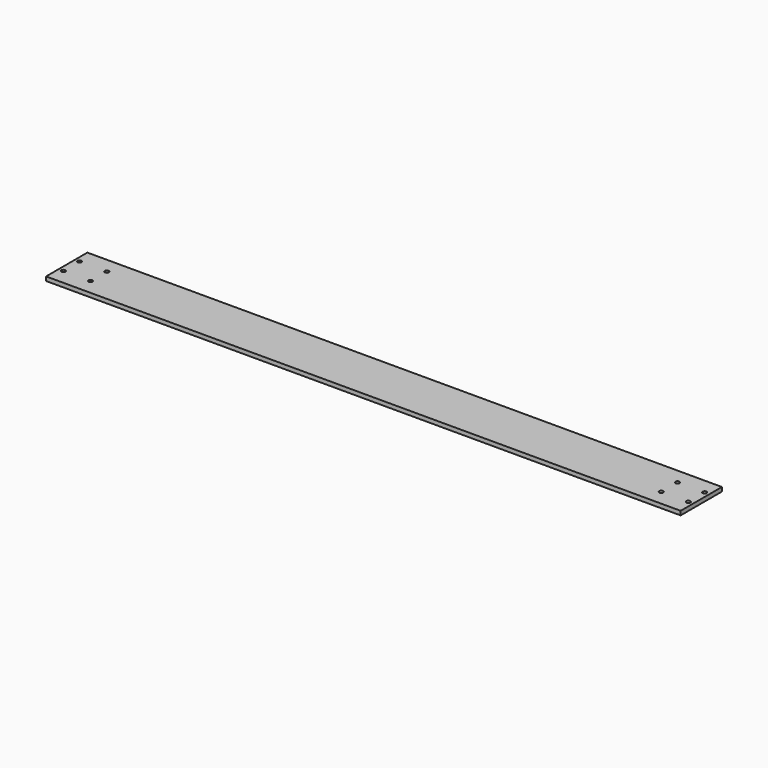
from build123d import *

# Parameters (mm, degrees)
F0_W     = 467
F0_H     = 38
F1_DEPTH = 3
F2_D     = 3


# Not quite as in the source:
# - a feature names something its author has since deleted; it is built from what else it names


with BuildPart() as f1:
    # F0 (on Top) → F1 (new body)
    with BuildSketch(Plane.XY):
        Rectangle(F0_W, F0_H)
    extrude(amount=F1_DEPTH)

    # F2 (through all)
    with Locations(Plane(origin=(0, 0, 0), x_dir=(1, 0, 0), z_dir=(0, 0, -1))):
        with Locations((-230, -7.5), (-210, -7.5), (-210, 7.5), (-230, 7.5), (210, -7.5), (230, -7.5), (230, 7.5), (210, 7.5)):
            Hole(F2_D / 2)


solid = f1.part
